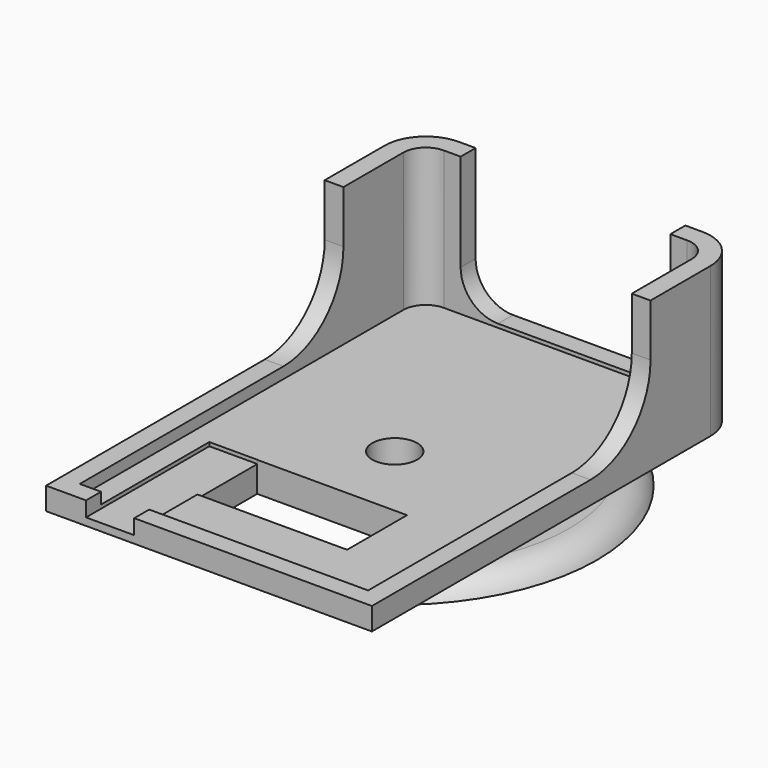
from build123d import *

# Parameters (mm, degrees)
F0_R      = 27
F0_R_2    = 3
F1_DEPTH  = 2.5
F2_W      = 25
F2_H      = 7
F2_R      = 0.3
F2_R_2    = 3
F3_DEPTH  = 1
F5_R      = 3
F6_DEPTH  = 1.5
F7_DEPTH  = 20
F8_W      = 36.5
F8_H      = 17
F8_W_2    = 10
F9_DEPTH  = 48.751
F10_W     = 28
F10_H     = 18
F11_DEPTH = 2.5
F12_R     = 10
F13_R     = 5
F14_W     = 20
F14_H     = 10
F15_DEPTH = 25
F16_W     = 6.433098577
F16_H     = 18.0739424974
F16_H_2   = 2.5
F17_DEPTH = 2


# Not quite as in the source:
# - a fillet or chamfer that OpenCascade refuses, or shapes differently, is made with other operations: its cross-section is extruded or revolved along the edge and cut away or added


with BuildPart() as f1:
    # F0 (on Top) → F1 (new body)
    with BuildSketch(Plane.XY):
        Circle(F0_R)
        Circle(F0_R_2, mode=Mode.SUBTRACT)
    extrude(amount=-F1_DEPTH)

    # F4: fillet of radius 4 on 1 edges, made by hand

    # F4_s1 → F4_t2 (revolve, cut)
    with BuildSketch(Plane.XZ):
        with BuildLine():
            ThreePointArc((27, -2.5), (25.527968734, -0.6833752096), (23.2919007565, 0))
            Line((23.2919007565, 0), (27, 0))
            Line((27, 0), (27, -2.5))
        make_face()
    revolve(axis=Axis((0, 0, 0), (0, 0, 1)), mode=Mode.SUBTRACT)

    # F5 (on face) → F6 (join)
    with BuildSketch(Plane.XY):
        with BuildLine():
            Line((-19.25, -28.5), (19.25, -28.5))
            Line((19.25, -28.5), (19.25, -13.1129760486))
            ThreePointArc((19.25, -13.1129760486), (0, -23.2919007565), (-19.25, -13.1129760486))
            Line((-19.25, -13.1129760486), (-19.25, -28.5))
        make_face()
        with BuildLine():
            ThreePointArc((-19.25, -13.1129760486), (0, -23.2919007565), (19.25, -13.1129760486))
            Line((19.25, -13.1129760486), (19.25, 13.1129760486))
            ThreePointArc((19.25, 13.1129760486), (0, 23.2919007565), (-19.25, 13.1129760486))
            Line((-19.25, 13.1129760486), (-19.25, -13.1129760486))
        make_face()
        Circle(F5_R, mode=Mode.SUBTRACT)
        with BuildLine():
            ThreePointArc((-19.25, 13.1129760486), (0, 23.2919007565), (19.25, 13.1129760486))
            Line((19.25, 13.1129760486), (19.25, 25.5))
            ThreePointArc((19.25, 25.5), (18.3713203436, 27.6213203436), (16.25, 28.5))
            Line((16.25, 28.5), (-16.25, 28.5))
            ThreePointArc((-16.25, 28.5), (-18.3713203436, 27.6213203436), (-19.25, 25.5))
            Line((-19.25, 25.5), (-19.25, 13.1129760486))
        make_face()
    extrude(amount=F6_DEPTH)

    # F5 (on face) → F7 (join)
    with BuildSketch(Plane.XY):
        with BuildLine():
            ThreePointArc((21.75, 25.5), (20.1390872965, 29.3890872965), (16.25, 31))
            Line((16.25, 31), (-16.25, 31))
            ThreePointArc((-16.25, 31), (-20.1390872965, 29.3890872965), (-21.75, 25.5))
            Line((-21.75, 25.5), (-21.75, -31))
            Line((-21.75, -31), (21.75, -31))
            Line((21.75, -31), (21.75, 25.5))
        make_face()
        with BuildLine():
            Line((19.25, 25.5), (19.25, -28.5))
            Line((19.25, -28.5), (-19.25, -28.5))
            Line((-19.25, -28.5), (-19.25, 25.5))
            ThreePointArc((-19.25, 25.5), (-18.3713203436, 27.6213203436), (-16.25, 28.5))
            Line((-16.25, 28.5), (16.25, 28.5))
            ThreePointArc((16.25, 28.5), (18.3713203436, 27.6213203436), (19.25, 25.5))
        make_face(mode=Mode.SUBTRACT)
    extrude(amount=F7_DEPTH)

    # F8 (on face) → F9 (cut, through all)
    with BuildSketch(Plane(origin=(-21.75, 0, 0), x_dir=(0, -1, 0), z_dir=(-1, 0, 0))):
        with Locations((2.75, 11.5)):
            Rectangle(F8_W, F8_H)
        with Locations((26, 11.5)):
            Rectangle(F8_W_2, F8_H)
    extrude(amount=-F9_DEPTH, mode=Mode.SUBTRACT)

    # F10 (on face) → F11 (cut)
    with BuildSketch(Plane(origin=(0, 31, 0), x_dir=(-1, 0, 0), z_dir=(0, 1, 0))):
        with Locations((0, 11)):
            Rectangle(F10_W, F10_H)
    extrude(amount=-F11_DEPTH, mode=Mode.SUBTRACT)

    # F12
    f12_edges = [f1.edges().sort_by_distance(p)[0] for p in [
        (-20.5, 15.5, 3),
        (20.5, 15.5, 3),
    ]]
    fillet(f12_edges, radius=F12_R)

    # F13
    f13_edges = [f1.edges().sort_by_distance(p)[0] for p in [
        (14, 29.75, 2),
        (-14, 29.75, 2),
    ]]
    fillet(f13_edges, radius=F13_R)

    # F14 (on face) → F15 (cut)
    with BuildSketch(Plane(origin=(0, 0, -2.5), x_dir=(1, 0, 0), z_dir=(0, 0, -1))):
        with Locations((0, 15.4472477734)):
            Rectangle(F14_W, F14_H)
    extrude(amount=-F15_DEPTH, mode=Mode.SUBTRACT)

    # F16 (on face) → F17 (cut)
    with BuildSketch(Plane.XY.offset(3)):
        with Locations((-13.1989442743, -19.4630287513)):
            Rectangle(F16_W, F16_H)
        with Locations((-13.1989442743, -29.75)):
            Rectangle(F16_W, F16_H_2)
    extrude(amount=-F17_DEPTH, mode=Mode.SUBTRACT)


with BuildPart() as f3:
    # F2 (on face) → F3 (new body)
    with BuildSketch(Plane(origin=(0, 0, -2.5), x_dir=(1, 0, 0), z_dir=(0, 0, -1))):
        Rectangle(F2_W, F2_H)
        with Locations((-11.5, 0)):
            Circle(F2_R, mode=Mode.SUBTRACT)
        with Locations((-6.5, 0)):
            Circle(F2_R, mode=Mode.SUBTRACT)
        Circle(F2_R_2, mode=Mode.SUBTRACT)
        with Locations((6.5, 0)):
            Circle(F2_R, mode=Mode.SUBTRACT)
        with Locations((11.5, 0)):
            Circle(F2_R, mode=Mode.SUBTRACT)
    extrude(amount=F3_DEPTH)


solid = Compound([f1.part, f3.part])
